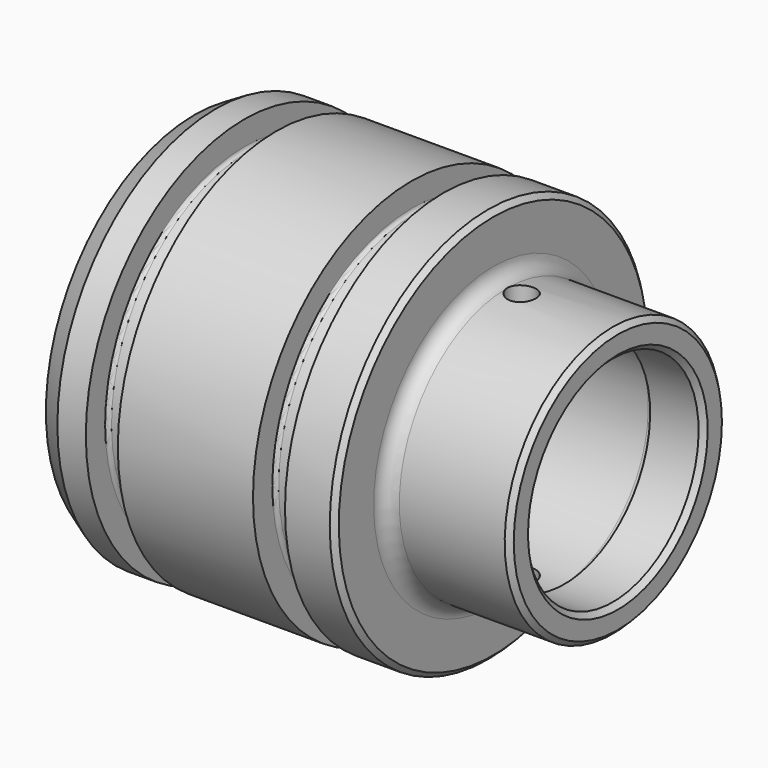
from build123d import *

# Parameters (mm, degrees)
F2_R     = 3.175
F4_R     = 0.79375
F5_R     = 3.175
F6_DEPTH = 50.8


# Not quite as in the source:
# - a fillet or chamfer that OpenCascade refuses, or shapes differently, is made with other operations: its cross-section is extruded or revolved along the edge and cut away or added


with BuildPart() as f1:
    # F0 (on Front) → F1 (revolve)
    with BuildSketch(Plane.XZ):
        Polygon((0, 25.0620320151), (1.1225320151, 23.9395), (15.875, 23.9395), (15.875, 27.6225), (19.05, 27.6225), (19.05, 23.9395), (28.575, 23.9395), (28.575, 27.6225), (31.75, 27.6225), (31.75, 23.9395), (47.625, 23.9395), (47.625, 25.4), (82.55, 25.4), (82.55, 23.9395), (93.3674679849, 23.9395), (94.49, 25.0620320151), (94.49, 29.0399679849), (93.3674679849, 30.1625), (66.675, 30.1625), (66.675, 43.0734679849), (65.5524679849, 44.196), (55.5625, 44.196), (55.5625, 38.0238), (48.4251, 38.0238), (48.4251, 44.196), (18.2499, 44.196), (18.2499, 38.0238), (11.1125, 38.0238), (11.1125, 44.196), (4.7625, 44.196), (0, 41.446369343), align=None)
    revolve(axis=Axis((55.6648539445, 0, 0), (1, 0, 0)))

    # F2
    f2_edges = [f1.edges().sort_by_distance(p)[0] for p in [
        (66.675, 0, -30.1625),
    ]]
    fillet(f2_edges, radius=F2_R)

    # F3: fillet of radius 1.5875 on 2 edges, made by hand

    # F3_s1 → F3_t2 (revolve)
    with BuildSketch(Plane.XZ):
        with BuildLine():
            ThreePointArc((49.2074118459, 25.4), (48.1307169611, 24.97906949), (47.625, 23.9395))
            Line((47.625, 23.9395), (47.625, 25.4))
            Line((47.625, 25.4), (49.2074118459, 25.4))
        make_face()
    revolve(axis=Axis((47.625, 0, 0), (1, 0, 0)))

    # F3_s3 → F3_t4 (revolve)
    with BuildSketch(Plane.XZ):
        with BuildLine():
            ThreePointArc((82.55, 23.9395), (82.0442830389, 24.97906949), (80.9675881541, 25.4))
            Line((80.9675881541, 25.4), (82.55, 25.4))
            Line((82.55, 25.4), (82.55, 23.9395))
        make_face()
    revolve(axis=Axis((82.55, 0, 0), (1, 0, 0)))

    # F4
    f4_edges = [f1.edges().sort_by_distance(p)[0] for p in [
        (18.2499, 0, -38.0238),
        (55.5625, 0, -38.0238),
        (19.05, 0, -27.6225),
        (31.75, 0, -27.6225),
        (15.875, 0, -27.6225),
        (28.575, 0, -27.6225),
        (11.1125, 0, -38.0238),
        (48.4251, 0, -38.0238),
    ]]
    fillet(f4_edges, radius=F4_R)

    # F5 (on Top) → F6 (cut, symmetric)
    with BuildSketch(Plane.XY):
        with Locations((73.025, 0)):
            Circle(F5_R)
    extrude(amount=F6_DEPTH, both=True, mode=Mode.SUBTRACT)


solid = f1.part
